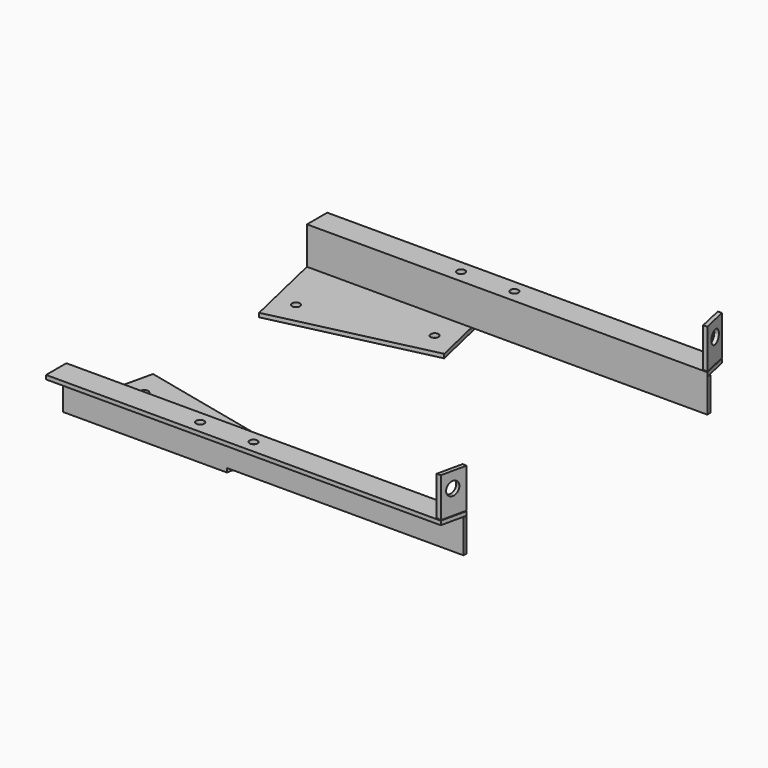
from build123d import *

# Parameters (mm, degrees)
F0_W        = 300
F0_H        = 16
F0_H_2      = 3
F1_DEPTH    = 3
F3_DEPTH    = 3.001
F5_DEPTH    = 30
F6_T1_DEPTH = 45.4466987362
F8_DEPTH    = 292.889802136
F10_DEPTH   = 25
F11_R       = 3
F12_DEPTH   = 3
F4_R        = 3
F13_DEPTH   = 31.001


# Not quite as in the source:
# - a fillet or chamfer that OpenCascade refuses, or shapes differently, is made with other operations: its cross-section is extruded or revolved along the edge and cut away or added


with BuildPart() as f1:
    # F0 (on Top) → F1 (new body)
    with BuildSketch(Plane.XY):
        with Locations((31.376008536, 23.679145366)):
            Rectangle(F0_W, F0_H)
        with Locations((31.376008536, 14.179145366)):
            Rectangle(F0_W, F0_H_2)
    extrude(amount=F1_DEPTH)

    # F2 (on face) → F3 (cut, through all)
    with BuildSketch(Plane.XY.offset(3)):
        Polygon((181.376008536, 31.679145366), (177.1638099458, 31.679145366), (181.376008536, 12.679145366), align=None)
    extrude(amount=-F3_DEPTH, mode=Mode.SUBTRACT)

    # F0 (on Top) → F10 (join)
    with BuildSketch(Plane.XY):
        with Locations((31.376008536, 14.179145366)):
            Rectangle(F0_W, F0_H_2)
    extrude(amount=-F10_DEPTH)

    # F11 (on face) → F12 (join)
    with BuildSketch(Plane(origin=(0, 0, -25), x_dir=(1, 0, 0), z_dir=(0, 0, -1))):
        Polygon((-104.0779183868, 50.3268192335), (-118.623991464, -12.679145366), (4.7014701045, -12.679145366), (13.0069077049, 23.2956572255), align=None)
        with Locations((-5.8458569022, 8.6824761846)):
            Circle(F11_R, mode=Mode.SUBTRACT)
        with Locations((-93.5391627328, 28.9280710755)):
            Circle(F11_R, mode=Mode.SUBTRACT)
        Polygon((4.7014701045, -12.679145366), (-118.623991464, -12.679145366), (-118.623991464, -15.679145366), (4.0088655312, -15.679145366), align=None)
    extrude(amount=F12_DEPTH)

    # F4 (on face) → F13 (cut, through all)
    with BuildSketch(Plane.XY.offset(3)):
        with Locations((29.2699092409, 22.179145366)):
            Circle(F4_R)
        with Locations((-10.7300907591, 22.179145366)):
            Circle(F4_R)
    extrude(amount=-F13_DEPTH, mode=Mode.SUBTRACT)


with BuildPart() as f5:
    # F4 (on face) → F5 (new body)
    with BuildSketch(Plane.XY.offset(3)):
        Polygon((177.1638099458, 31.679145366), (174.0909714028, 31.679145366), (178.3031699931, 12.679145366), (181.376008536, 12.679145366), align=None)
    extrude(amount=F5_DEPTH)

    # F6: chamfer of 5 x 0.8816349035 on 1 edges, made by hand

    # F6_s2 → F6_t1 (cut)
    with BuildSketch(Plane(origin=(-1.3507421597, 6.0928041458, 0), x_dir=(0, 0, 1), z_dir=(0.2164396139, -0.9762960071, 0))):
        Polygon((3.8816349035, -176.8209422491), (3, -181.8209422491), (3, -176.8209422491), align=None)
    extrude(amount=F6_T1_DEPTH, mode=Mode.SUBTRACT)

    # F7 (on face) → F8 (cut, through all)
    with BuildSketch(Plane(origin=(175.5584679144, 38.9203753184, 0), x_dir=(-0.2164396139, 0.9762960071, 0), z_dir=(0.9762960071, 0.2164396139, 0))):
        with BuildLine():
            ThreePointArc((-11.4232179523, 21.3526539614), (-19.6925906243, 25.1356689404), (-17.1476988847, 16.4054196453))
            ThreePointArc((-17.1476988847, 16.4054196453), (-13.1538452802, 17.5696389824), (-11.4232179523, 21.3526539614))
        make_face()
    extrude(amount=-F8_DEPTH, mode=Mode.SUBTRACT)


with BuildPart() as f14_1:
    # F14: instance of F1
    add(f1.part.mirror(Plane.XZ.offset(100)))


with BuildPart() as f14_2:
    # F14: instance of F5
    add(f5.part.mirror(Plane.XZ.offset(100)))


solid = Compound([f1.part, f5.part, f14_1.part, f14_2.part])
